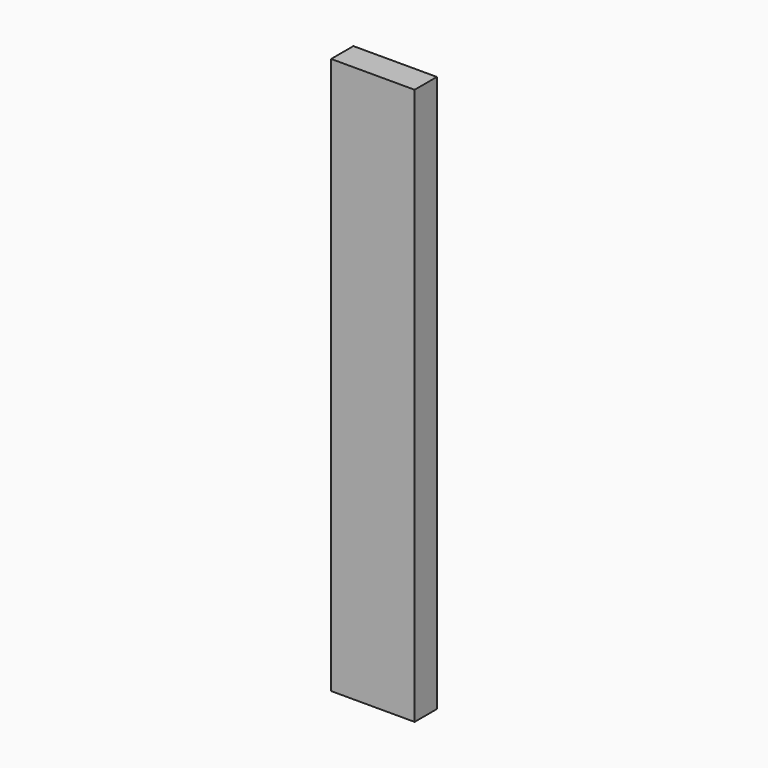
from build123d import *

# Parameters (mm, degrees)
F1_W     = 76.2
F1_H     = 508
F2_DEPTH = 25.4


# Not quite as in the source:
# - a variable given as a bare number and used for a length is read in inches; the dataset says mm whatever the document's units were


with BuildPart() as f2:
    # F1 (on Front) → F2 (new body)
    with BuildSketch(Plane.XZ):
        with Locations((38.1, -254)):
            Rectangle(F1_W, F1_H)
    extrude(amount=F2_DEPTH)


solid = f2.part
